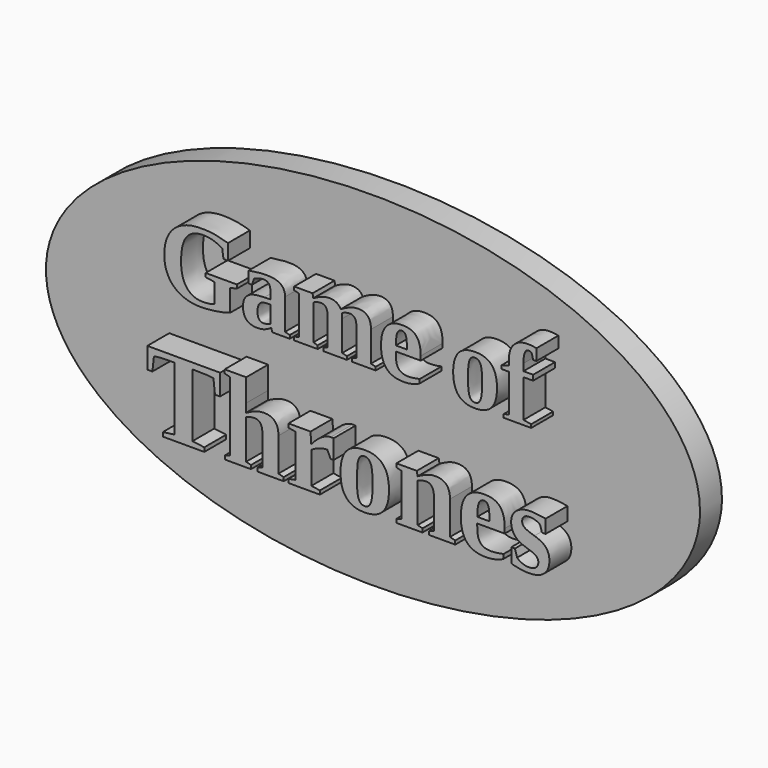
from build123d import *

# Parameters (mm, degrees)
F2_DEPTH       = 12.7
F1_TEXT_SIZE   = 47.9245283019
F1_TEXT_SIZE_2 = 53.0017823762
F3_DEPTH       = 25.4


# Not quite as in the source:
# - Text() gives the source's letters only with a copy of the font that has no kerning and outlines rounded to 1/6400 em; it was checked with that copy


with BuildPart() as f2:
    # F0 (on Front) → F2 (new body)
    with BuildSketch(Plane.XZ):
        with BuildLine():
            add(Edge.make_bspline(
                [(151.5751481056, 0), (151.5751481056, 138.0313373608), (-75.7875740528, 69.0156686804), (-303.1502962112, 0), (-75.7875740528, -69.0156686804), (151.5751481056, -138.0313373608), (151.5751481056, 0)],
                knots=[0, 0, 0, 2.0943951024, 2.0943951024, 4.1887902048, 4.1887902048, 6.2831853072, 6.2831853072, 6.2831853072], degree=2, weights=[1, 0.5, 1, 0.5, 1, 0.5, 1]))
        make_face()
    extrude(amount=F2_DEPTH)

    # F1 (on Front) → F3 (join)
    with BuildSketch(Plane.XZ):
        with Locations((-88.9, 16.9265393988)):
            Text('Game of', F1_TEXT_SIZE, font='Tinos', font_style=FontStyle.BOLD, text_align=(TextAlign.LEFT, TextAlign.BOTTOM))
        with Locations((-95.25, -42.1331403296)):
            Text('Thrones', F1_TEXT_SIZE_2, font='Tinos', font_style=FontStyle.BOLD, text_align=(TextAlign.LEFT, TextAlign.BOTTOM))
    extrude(amount=F3_DEPTH)


solid = f2.part
